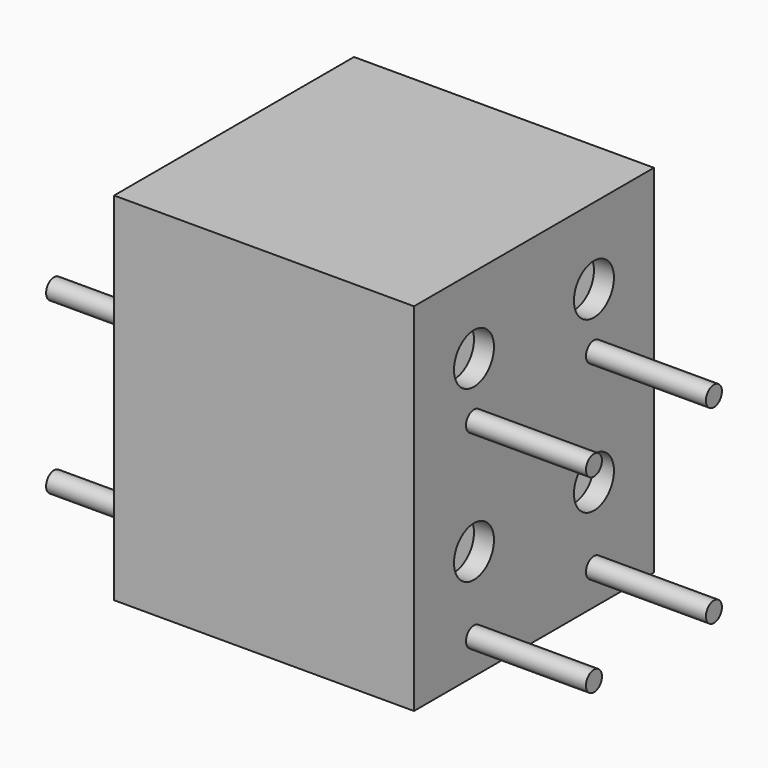
from build123d import *

# Parameters (mm, degrees)
F0_W      = 177.8
F0_H      = 177.8
F1_DEPTH  = 12.7
F2_W      = 177.8
F2_H      = 203.2
F3_DEPTH  = 12.7
F4_W      = 165.1
F4_H      = 203.2
F5_DEPTH  = 12.7
F6_W      = 165.1
F6_H      = 12.7
F7_DEPTH  = 165.1
F8_W      = 12.7
F8_H      = 76.2
F8_W_2    = 76.2
F8_H_2    = 12.7
F9_DEPTH  = 203.2
F10_W     = 76.2
F10_H     = 95.25
F11_DEPTH = 12.7
F12_W     = 76.2
F12_H     = 95.25
F13_DEPTH = 12.7
F15_D     = 31.75
F15_DEPTH = 12.7
F15_TIP   = 9.5386623271
F17_D     = 31.75
F17_DEPTH = 12.7
F17_TIP   = 9.5386623271
F18_W     = 190.5
F18_H     = 190.5
F19_DEPTH = 10.414
F14_R     = 6.35
F20_DEPTH = 76.2
F16_R     = 6.35
F21_DEPTH = 76.2


with BuildPart() as f1:
    # F0 (on Top) → F1 (new body)
    with BuildSketch(Plane.XY):
        with Locations((13.2262037635, 56.5882699132)):
            Rectangle(F0_W, F0_H)
    extrude(amount=F1_DEPTH)

    # F2 (on face) → F3 (join)
    with BuildSketch(Plane.YZ.offset(102.1262037635)):
        with Locations((56.5882699132, 114.3)):
            Rectangle(F2_W, F2_H)
    extrude(amount=-F3_DEPTH)

    # F4 (on face) → F5 (join)
    with BuildSketch(Plane(origin=(0, 145.4882699132, 0), x_dir=(-1, 0, 0), z_dir=(0, 1, 0))):
        with Locations((-6.8762037635, 114.3)):
            Rectangle(F4_W, F4_H)
    extrude(amount=-F5_DEPTH)

    # F6 (on face) → F7 (join, through all)
    with BuildSketch(Plane(origin=(89.4262037635, 0, 0), x_dir=(0, -1, 0), z_dir=(-1, 0, 0))):
        with Locations((-50.2382699132, 114.3)):
            Rectangle(F6_W, F6_H)
    extrude(amount=F7_DEPTH)

    # F8 (on face) → F9 (join, through all)
    with BuildSketch(Plane.XY.offset(12.7)):
        with Locations((6.8762037635, 94.6882699132)):
            Rectangle(F8_W, F8_H)
        with Locations((-37.5737962365, 50.2382699132)):
            Rectangle(F8_W_2, F8_H_2)
        with Locations((6.8762037635, 50.2382699132)):
            Rectangle(F8_W, F8_H_2)
        with Locations((6.8762037635, 5.7882699132)):
            Rectangle(F8_W, F8_H)
        with Locations((51.3262037635, 50.2382699132)):
            Rectangle(F8_W_2, F8_H_2)
    extrude(amount=F9_DEPTH)

    # F10 (on face) → F11 (join)
    with BuildSketch(Plane(origin=(-75.6737962365, 0, 0), x_dir=(0, -1, 0), z_dir=(-1, 0, 0))):
        Polygon((-132.7882699132, 215.9), (-145.4882699132, 215.9), (-145.4882699132, 0), (32.3117300868, 0), (32.3117300868, 12.7), (-43.8882699132, 12.7), (-43.8882699132, 107.95), (32.3117300868, 107.95), (32.3117300868, 120.65), (-43.8882699132, 120.65), (-43.8882699132, 215.9), (-56.5882699132, 215.9), (-56.5882699132, 120.65), (-132.7882699132, 120.65), align=None)
        with Locations((-94.6882699132, 60.325)):
            Rectangle(F10_W, F10_H, mode=Mode.SUBTRACT)
        with Locations((-94.6882699132, 168.275)):
            Rectangle(F10_W, F10_H)
        with Locations((-5.7882699132, 168.275)):
            Rectangle(F10_W, F10_H)
        with Locations((-5.7882699132, 60.325)):
            Rectangle(F10_W, F10_H)
        with Locations((-94.6882699132, 60.325)):
            Rectangle(F10_W, F10_H)
    extrude(amount=F11_DEPTH)

    # F12 (on face) → F13 (join)
    with BuildSketch(Plane.XZ.offset(32.3117300868)):
        Polygon((-75.6737962365, 215.9), (-88.3737962365, 215.9), (-88.3737962365, 0), (102.1262037635, 0), (102.1262037635, 215.9), (89.4262037635, 215.9), (89.4262037635, 120.65), (13.2262037635, 120.65), (13.2262037635, 215.9), (0.5262037635, 215.9), (0.5262037635, 120.65), (-75.6737962365, 120.65), align=None)
        with Locations((-37.5737962365, 60.325)):
            Rectangle(F12_W, F12_H, mode=Mode.SUBTRACT)
        with Locations((51.3262037635, 60.325)):
            Rectangle(F12_W, F12_H, mode=Mode.SUBTRACT)
        with Locations((-37.5737962365, 168.275)):
            Rectangle(F12_W, F12_H)
        with Locations((51.3262037635, 168.275)):
            Rectangle(F12_W, F12_H)
        with Locations((-37.5737962365, 60.325)):
            Rectangle(F12_W, F12_H)
        with Locations((51.3262037635, 60.325)):
            Rectangle(F12_W, F12_H)
    extrude(amount=F13_DEPTH)

    # F15
    with Locations(Plane.YZ.offset(102.1262037635)):
        with Locations((2.6132699132, 177.8), (97.8632699132, 177.8), (2.6132699132, 69.85), (97.8632699132, 69.85)):
            Hole(F15_D / 2, depth=F15_DEPTH)
            with Locations((0, 0, -(F15_DEPTH + F15_TIP / 2))):  # 118° drill point
                Cone(0, F15_D / 2, F15_TIP, mode=Mode.SUBTRACT)

    # F17
    with Locations(Plane(origin=(-88.3737962365, 0, 0), x_dir=(0, -1, 0), z_dir=(-1, 0, 0))):
        with Locations((-97.8632699132, 177.8), (-2.6132699132, 177.8), (-97.8632699132, 69.85), (-2.6132699132, 69.85)):
            Hole(F17_D / 2, depth=F17_DEPTH)
            with Locations((0, 0, -(F17_DEPTH + F17_TIP / 2))):  # 118° drill point
                Cone(0, F17_D / 2, F17_TIP, mode=Mode.SUBTRACT)

    # F18 (on face) → F19 (join)
    with BuildSketch(Plane.XY.offset(215.9)):
        with Locations((6.8762037635, 50.2382699132)):
            Rectangle(F18_W, F18_H)
    extrude(amount=F19_DEPTH)

    # F14 (on face) → F20 (join)
    with BuildSketch(Plane.YZ.offset(102.1262037635)):
        with Locations((2.6132699132, 142.875)):
            Circle(F14_R)
        with Locations((2.6132699132, 22.225)):
            Circle(F14_R)
        with Locations((97.8632699132, 142.875)):
            Circle(F14_R)
        with Locations((97.8632699132, 22.225)):
            Circle(F14_R)
    extrude(amount=F20_DEPTH)

    # F16 (on face) → F21 (join)
    with BuildSketch(Plane(origin=(-88.3737962365, 0, 0), x_dir=(0, -1, 0), z_dir=(-1, 0, 0))):
        with Locations((-97.8632699132, 130.175)):
            Circle(F16_R)
        with Locations((-97.8632699132, 22.225)):
            Circle(F16_R)
        with Locations((-2.6132699132, 130.175)):
            Circle(F16_R)
        with Locations((-2.6132699132, 22.225)):
            Circle(F16_R)
    extrude(amount=F21_DEPTH)


solid = f1.part
